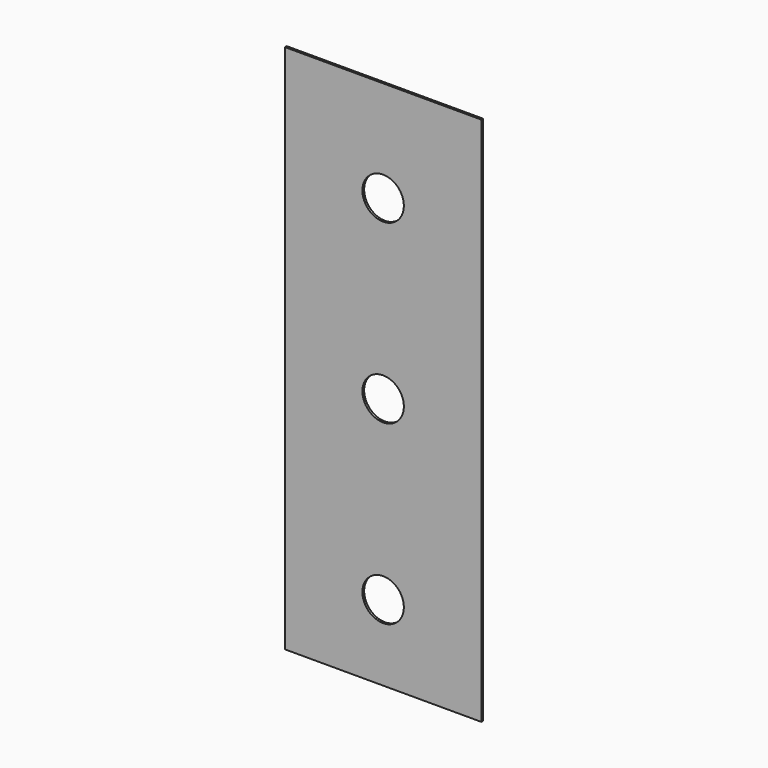
from build123d import *

# Parameters (mm, degrees)
F0_W     = 286
F0_H     = 771.5
F0_R     = 30.1625
F1_DEPTH = 3.175


# Not quite as in the source:
# - a length typed as a fraction of an inch, garbled in the dataset ("3 / 203.2 mm" for 3/8 in), is restored


with BuildPart() as f1:
    # F0 (on Front) → F1 (new body)
    with BuildSketch(Plane.XZ):
        with Locations((143, 385.75)):
            Rectangle(F0_W, F0_H)
        with Locations((143, 110.1625)):
            Circle(F0_R, mode=Mode.SUBTRACT)
        with Locations((143, 367.3291666667)):
            Circle(F0_R, mode=Mode.SUBTRACT)
        with Locations((143, 624.4958333333)):
            Circle(F0_R, mode=Mode.SUBTRACT)
    extrude(amount=F1_DEPTH)


solid = f1.part
